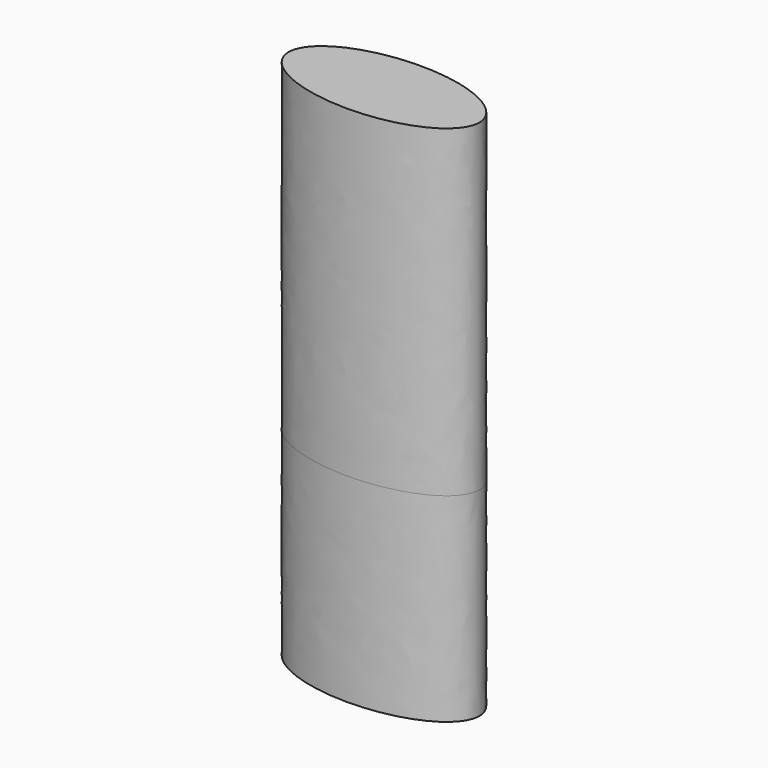
from build123d import *

# Parameters (mm, degrees)
F1_DEPTH      = 112.63112
F1_DEPTH_BACK = 69.3044


# Not quite as in the source:
# - the program builds the solid bodies; features that only make, move or delete a surface that nothing else refers to are left out


with BuildPart() as f1:
    # F0 (on Top) → F1 (new body, two sides)
    with BuildSketch(Plane.XY) as f1_sk:
        with BuildLine():
            add(Edge.make_bspline(
                [(33.2171469927, 0), (33.2171469927, 27.84506076), (-16.6085734963, 13.92253038), (-66.4342939854, 0), (-16.6085734963, -13.92253038), (33.2171469927, -27.84506076), (33.2171469927, 0)],
                knots=[0, 0, 0, 2.0943951024, 2.0943951024, 4.1887902048, 4.1887902048, 6.2831853072, 6.2831853072, 6.2831853072], degree=2, weights=[1, 0.5, 1, 0.5, 1, 0.5, 1]))
        make_face()
    extrude(amount=F1_DEPTH)
    extrude(f1_sk.sketch, amount=-F1_DEPTH_BACK)


solid = f1.part
